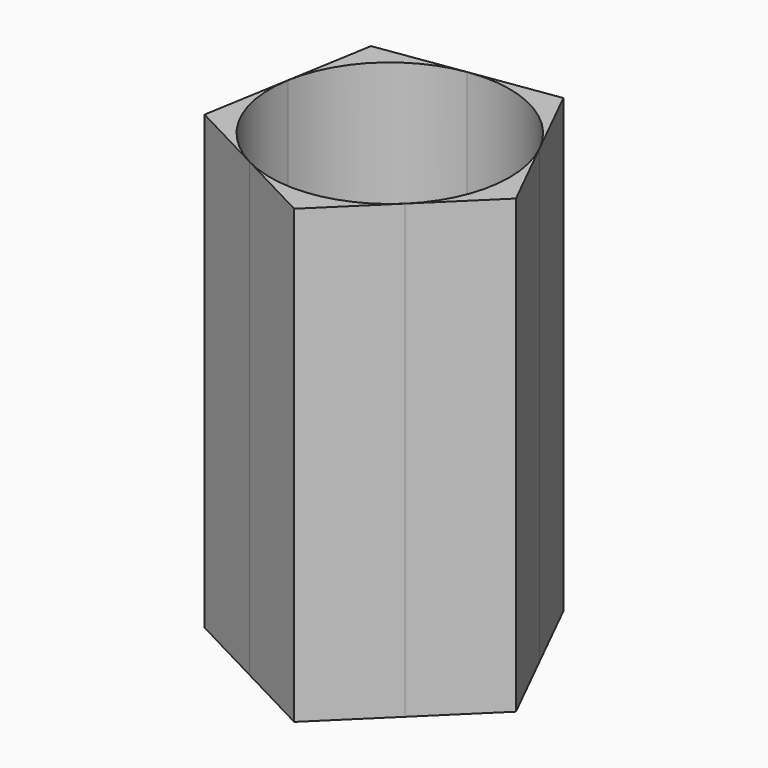
from build123d import *

# Parameters (mm, degrees)
F6_DEPTH = 183
F7_R     = 48
F8_DEPTH = 12


# Not quite as in the source:
# - a feature of the source that left no trace in its solid (it failed there, or was rolled back) is left out


with BuildPart() as f6:
    # F5 (on face) → F6 (new body)
    with BuildSketch(Plane.XY):
        with BuildLine():
            ThreePointArc((37.2800312122, -34.6786276575), (10.4193238865, -47.9901283759), (-19.135748604, -42.9710308984))
            Line((-19.135748604, -42.9710308984), (12.0845335159, -59.319060862))
            Line((12.0845335159, -59.319060862), (37.2800312122, -34.6786276575))
        make_face()
    extrude(amount=F6_DEPTH)


with BuildPart() as f6b:
    # F5 (on face) → F6, piece 2 (new body)
    with BuildSketch(Plane.XY):
        with BuildLine():
            ThreePointArc((-19.135748604, -42.9710308984), (-40.0961528093, -21.538460152), (-44.4557270426, 8.1210702852))
            Line((-44.4557270426, 8.1210702852), (-50.3560297098, -26.6230014659))
            Line((-50.3560297098, -26.6230014659), (-19.135748604, -42.9710308984))
        make_face()
    extrude(amount=F6_DEPTH)


with BuildPart() as f6c:
    # F5 (on face) → F6, piece 3 (new body)
    with BuildSketch(Plane.XY):
        with BuildLine():
            ThreePointArc((-44.4557270426, 8.1210702852), (-30.5492623338, 34.6786277053), (-3.6885555549, 47.9901283027))
            Line((-3.6885555549, 47.9901283027), (-38.555424539, 42.8651410735))
            Line((-38.555424539, 42.8651410735), (-44.4557270426, 8.1210702852))
        make_face()
    extrude(amount=F6_DEPTH)


with BuildPart() as f6d:
    # F5 (on face) → F6, piece 4 (new body)
    with BuildSketch(Plane.XY):
        with BuildLine():
            Line((46.8269215589, 21.5384603135), (31.17831377, 53.1151155819))
            Line((31.17831377, 53.1151155819), (-3.6885555549, 47.9901283027))
            ThreePointArc((-3.6885555549, 47.9901283027), (25.8665170053, 42.9710311227), (46.8269215589, 21.5384603135))
        make_face()
    extrude(amount=F6_DEPTH)


with BuildPart() as f6e:
    # F5 (on face) → F6, piece 5 (new body)
    with BuildSketch(Plane.XY):
        with BuildLine():
            Line((62.4755290368, -10.0381943275), (46.8269215589, 21.5384603135))
            ThreePointArc((46.8269215589, 21.5384603135), (50.5932689153, 11.0606242686), (51.8711622521, 0))
            ThreePointArc((51.8711622521, 0), (48.0748174608, -18.8116208847), (37.2800312122, -34.6786276575))
            Line((37.2800312122, -34.6786276575), (62.4755290368, -10.0381943275))
        make_face()
    extrude(amount=F6_DEPTH)


with BuildPart() as f8:
    # F7 (on face) → F8 (new body)
    with BuildSketch(Plane.XY):
        with Locations((3.3653844148, 0)):
            Circle(F7_R)
    extrude(amount=F8_DEPTH)


solid = Compound([f6.part, f6b.part, f6c.part, f6d.part, f6e.part, f8.part])
